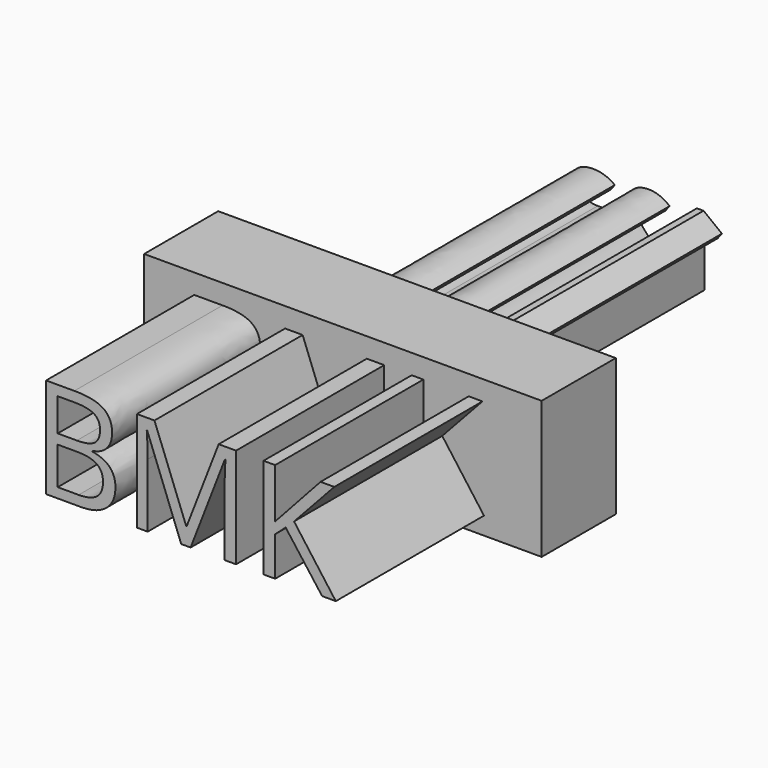
from build123d import *

# Parameters (mm, degrees)
F0_W         = 109.0458929539
F0_H         = 37.7005673945
F1_DEPTH     = 25.4
F3_TEXT_SIZE = 38.4569827778
F4_DEPTH     = 50.8
F5_TEXT_SIZE = 26.6819118729
F6_DEPTH     = 76.2


# Not quite as in the source:
# - Text() gives the source's letters only with a copy of the font that has no kerning and outlines rounded to 1/6400 em; it was checked with that copy


with BuildPart() as f1:
    # F0 (on Front) → F1 (new body)
    with BuildSketch(Plane.XZ):
        with Locations((54.5229464769, 18.8502836972)):
            Rectangle(F0_W, F0_H)
    extrude(amount=F1_DEPTH)

    # F3 (on face) → F4 (join)
    with BuildSketch(Plane.XZ.offset(25.4)):
        with Locations((9.9795965943, 4.8250965774)):
            Text('BMK', F3_TEXT_SIZE, font='Open Sans', text_align=(TextAlign.LEFT, TextAlign.BOTTOM))
    extrude(amount=F4_DEPTH)

    # F5 (on face) → F6 (join)
    with BuildSketch(Plane(origin=(0, 0, 0), x_dir=(-1, 0, 0), z_dir=(0, 1, 0))):
        with Locations((-79.6550139785, 11.2521322444)):
            Text('123', F5_TEXT_SIZE, font='Open Sans', text_align=(TextAlign.LEFT, TextAlign.BOTTOM))
    extrude(amount=F6_DEPTH)


solid = f1.part
